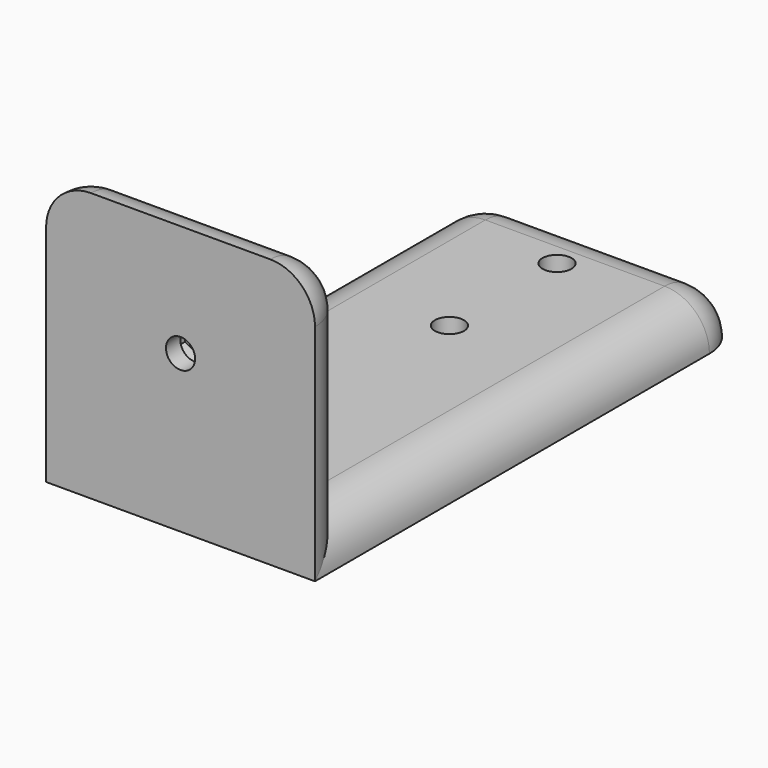
from build123d import *

# Parameters (mm, degrees)
F0_W     = 30
F0_H     = 60
F0_R     = 1.625
F1_DEPTH = 5
F2_W     = 5
F2_H     = 25
F3_DEPTH = 30
F4_R     = 1.625
F5_DEPTH = 25
F6_R     = 1.625
F7_DEPTH = 3
F8_R     = 4.99999


# Not quite as in the source:
# - a fillet or chamfer is up to 0.001 mm smaller than in the source, because OpenCascade refuses the exact size


with BuildPart() as f1:
    # F0 (on Top) → F1 (new body)
    with BuildSketch(Plane.XY):
        Rectangle(F0_W, F0_H)
        with Locations((0, 7.5)):
            Circle(F0_R, mode=Mode.SUBTRACT)
        with Locations((0, 22.5)):
            Circle(F0_R, mode=Mode.SUBTRACT)
    extrude(amount=F1_DEPTH)

    # F2 (on face) → F3 (join)
    with BuildSketch(Plane.YZ.offset(15)):
        with Locations((-27.5, 17.5)):
            Rectangle(F2_W, F2_H)
    extrude(amount=-F3_DEPTH)

    # F4 (on face) → F5 (cut)
    with BuildSketch(Plane(origin=(0, -25, 0), x_dir=(-1, 0, 0), z_dir=(0, 1, 0))):
        with Locations((0, 17.5)):
            Circle(F4_R)
    extrude(amount=-F5_DEPTH, mode=Mode.SUBTRACT)

    # F6 (on face) → F7 (cut)
    with BuildSketch(Plane(origin=(0, -25, 0), x_dir=(-1, 0, 0), z_dir=(0, 1, 0))):
        Polygon((3.5, 15.4792740578), (3.5, 19.5207259422), (0, 21.5414518843), (-3.5, 19.5207259422), (-3.5, 15.4792740578), (0, 13.4585481157), align=None)
        with Locations((0, 17.5)):
            Circle(F6_R, mode=Mode.SUBTRACT)
    extrude(amount=-F7_DEPTH, mode=Mode.SUBTRACT)

    # F8 (radius 5 in the source; OpenCascade refuses exactly that, so slightly less here)
    f8_edges = [f1.edges().sort_by_distance(p)[0] for p in [
        (0, 30, 5),
        (15, 30, 2.5),
        (-15, 30, 2.5),
        (15, 2.5, 5),
        (-15, 2.5, 5),
        (-15, -25, 17.5),
        (0, -25, 30),
        (15, -25, 17.5),
        (-15, -27.5, 30),
        (15, -27.5, 30),
    ]]
    fillet(f8_edges, radius=F8_R)


solid = f1.part
